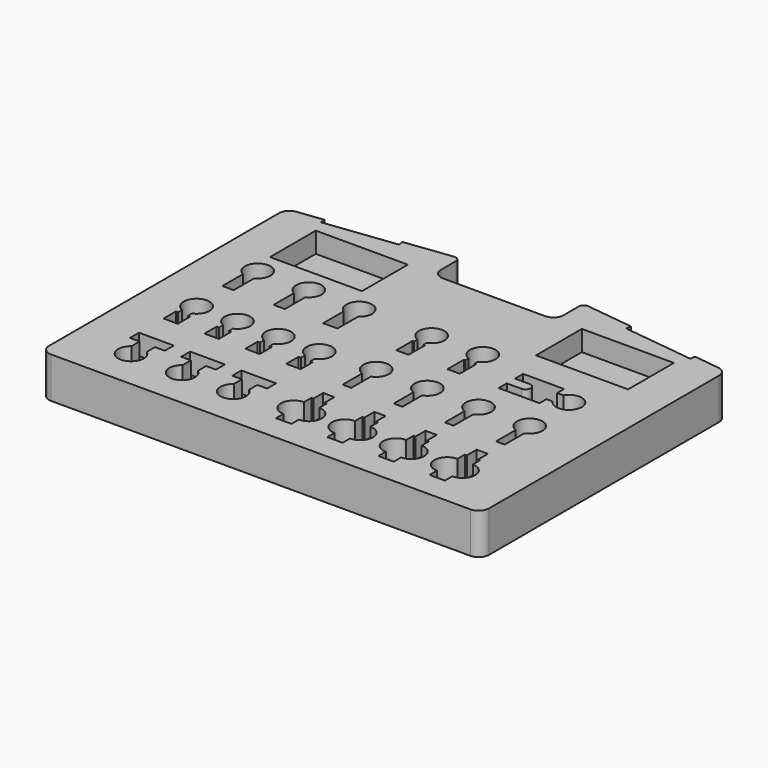
from build123d import *

# Parameters (mm, degrees)
F0_W     = 90
F0_H     = 56
F1_DEPTH = 20
F2_DEPTH = 20


# Not quite as in the source:
# - a feature names something its author has since deleted; it is built from what else it names


with BuildPart() as f1:
    # F0 (on Top) → F1 (new body)
    with BuildSketch(Plane.XY):
        with BuildLine():
            ThreePointArc((0, 10), (2.9289321881, 2.9289321881), (10, 0))
            Line((10, 0), (420, 0))
            ThreePointArc((420, 0), (427.0710678119, 2.9289321881), (430, 10))
            Line((430, 10), (430, 291.1509565045))
            ThreePointArc((430, 291.1509565045), (427.4888915944, 297.7779092497), (421.2166994626, 301.0766626465))
            Line((421.2166994626, 301.0766626465), (396.0936149327, 304.1562665566))
            Line((396.0936149327, 304.1562665566), (395.4852652014, 299.1934134856))
            Line((395.4852652014, 299.1934134856), (326.0053222072, 307.7103097236))
            Line((326.0053222072, 307.7103097236), (326.6136719385, 312.6731627946))
            Line((326.6136719385, 312.6731627946), (280.6083497313, 318.3125248716))
            ThreePointArc((280.6083497313, 318.3125248716), (276.6865236274, 317.0941175978), (275, 313.3496718006))
            Line((275, 313.3496718006), (275, 295))
            ThreePointArc((275, 295), (272.0710678119, 287.9289321881), (265, 285))
            Line((265, 285), (165, 285))
            ThreePointArc((165, 285), (157.9289321881, 287.9289321881), (155, 295))
            Line((155, 295), (155, 313.3496718006))
            ThreePointArc((155, 313.3496718006), (153.3134763726, 317.0941175978), (149.3916502687, 318.3125248716))
            Line((149.3916502687, 318.3125248716), (103.3863280615, 312.6731627946))
            Line((103.3863280615, 312.6731627946), (103.9946777928, 307.7103097236))
            Line((103.9946777928, 307.7103097236), (34.5147347986, 299.1934134856))
            Line((34.5147347986, 299.1934134856), (33.9063850673, 304.1562665566))
            Line((33.9063850673, 304.1562665566), (8.7833005374, 301.0766626465))
            ThreePointArc((8.7833005374, 301.0766626465), (2.5111084056, 297.7779092497), (0, 291.1509565045))
            Line((0, 291.1509565045), (0, 10))
        make_face()
        with BuildLine():
            Line((49.5, 59), (40, 59))
            Line((40, 59), (40, 70))
            Line((40, 70), (74, 70))
            Line((74, 70), (74, 59))
            Line((74, 59), (64.5, 59))
            Line((64.5, 59), (64.5, 49))
            ThreePointArc((64.5, 49), (57, 26.5), (49.5, 49))
            Line((49.5, 49), (49.5, 59))
        make_face(mode=Mode.SUBTRACT)
        with BuildLine():
            Line((99.5, 59), (90, 59))
            Line((90, 59), (90, 70))
            Line((90, 70), (124, 70))
            Line((124, 70), (124, 59))
            Line((124, 59), (114.5, 59))
            Line((114.5, 59), (114.5, 49))
            ThreePointArc((114.5, 49), (107, 26.5), (99.5, 49))
            Line((99.5, 49), (99.5, 59))
        make_face(mode=Mode.SUBTRACT)
        with BuildLine():
            Line((149.5, 59), (140, 59))
            Line((140, 59), (140, 70))
            Line((140, 70), (174, 70))
            Line((174, 70), (174, 59))
            Line((174, 59), (164.5, 59))
            Line((164.5, 59), (164.5, 49))
            ThreePointArc((164.5, 49), (157, 26.5), (149.5, 49))
            Line((149.5, 49), (149.5, 59))
        make_face(mode=Mode.SUBTRACT)
        with BuildLine():
            Line((54, 100), (40, 100))
            Line((40, 100), (40, 115))
            Line((40, 115), (42.25, 115))
            Line((42.25, 115), (42.25, 120))
            ThreePointArc((42.25, 120), (47, 144.0623310798), (51.75, 120))
            Line((51.75, 120), (51.75, 115))
            Line((51.75, 115), (54, 115))
            Line((54, 115), (54, 100))
        make_face(mode=Mode.SUBTRACT)
        with BuildLine():
            Line((94, 100), (80, 100))
            Line((80, 100), (80, 115))
            Line((80, 115), (82.25, 115))
            Line((82.25, 115), (82.25, 120))
            ThreePointArc((82.25, 120), (87, 144.0623310798), (91.75, 120))
            Line((91.75, 120), (91.75, 115))
            Line((91.75, 115), (94, 115))
            Line((94, 115), (94, 100))
        make_face(mode=Mode.SUBTRACT)
        with BuildLine():
            Line((134, 100), (120, 100))
            Line((120, 100), (120, 115))
            Line((120, 115), (122.25, 115))
            Line((122.25, 115), (122.25, 120))
            ThreePointArc((122.25, 120), (127, 144.0623310798), (131.75, 120))
            Line((131.75, 120), (131.75, 115))
            Line((131.75, 115), (134, 115))
            Line((134, 115), (134, 100))
        make_face(mode=Mode.SUBTRACT)
        with BuildLine():
            Line((174, 100), (160, 100))
            Line((160, 100), (160, 115))
            Line((160, 115), (162.25, 115))
            Line((162.25, 115), (162.25, 120))
            ThreePointArc((162.25, 120), (167, 144.0623310798), (171.75, 120))
            Line((171.75, 120), (171.75, 115))
            Line((171.75, 115), (174, 115))
            Line((174, 115), (174, 100))
        make_face(mode=Mode.SUBTRACT)
        with BuildLine():
            Line((225, 25), (210, 25))
            Line((210, 25), (210, 34))
            ThreePointArc((210, 34), (197.5, 46.5), (210, 59))
            Line((210, 59), (210, 68))
            Line((210, 68), (212, 68))
            Line((212, 68), (212, 80))
            Line((212, 80), (223, 80))
            Line((223, 80), (223, 68))
            Line((223, 68), (225, 68))
            Line((225, 68), (225, 59))
            ThreePointArc((225, 59), (237.5, 46.5), (225, 34))
            Line((225, 34), (225, 25))
        make_face(mode=Mode.SUBTRACT)
        with BuildLine():
            Line((275, 34), (275, 25))
            Line((275, 25), (260, 25))
            Line((260, 25), (260, 34))
            ThreePointArc((260, 34), (247.5, 46.5), (260, 59))
            Line((260, 59), (260, 68))
            Line((260, 68), (262, 68))
            Line((262, 68), (262, 80))
            Line((262, 80), (273, 80))
            Line((273, 80), (273, 68))
            Line((273, 68), (275, 68))
            Line((275, 68), (275, 59))
            ThreePointArc((275, 59), (287.5, 46.5), (275, 34))
        make_face(mode=Mode.SUBTRACT)
        with BuildLine():
            Line((325, 34), (325, 25))
            Line((325, 25), (310, 25))
            Line((310, 25), (310, 34))
            ThreePointArc((310, 34), (297.5, 46.5), (310, 59))
            Line((310, 59), (310, 68))
            Line((310, 68), (312, 68))
            Line((312, 68), (312, 80))
            Line((312, 80), (323, 80))
            Line((323, 80), (323, 68))
            Line((323, 68), (325, 68))
            Line((325, 68), (325, 59))
            ThreePointArc((325, 59), (337.5, 46.5), (325, 34))
        make_face(mode=Mode.SUBTRACT)
        with BuildLine():
            Line((375, 34), (375, 25))
            Line((375, 25), (360, 25))
            Line((360, 25), (360, 34))
            ThreePointArc((360, 34), (347.5, 46.5), (360, 59))
            Line((360, 59), (360, 68))
            Line((360, 68), (362, 68))
            Line((362, 68), (362, 80))
            Line((362, 80), (373, 80))
            Line((373, 80), (373, 68))
            Line((373, 68), (375, 68))
            Line((375, 68), (375, 59))
            ThreePointArc((375, 59), (387.5, 46.5), (375, 34))
        make_face(mode=Mode.SUBTRACT)
        with BuildLine():
            Line((223.5, 124), (223.5, 100))
            Line((223.5, 100), (215, 100))
            Line((215, 100), (215, 124))
            ThreePointArc((215, 124), (219.25, 148.2553179455), (223.5, 124))
        make_face(mode=Mode.SUBTRACT)
        with BuildLine():
            Line((273.5, 124), (273.5, 100))
            Line((273.5, 100), (265, 100))
            Line((265, 100), (265, 124))
            ThreePointArc((265, 124), (269.25, 148.2553179455), (273.5, 124))
        make_face(mode=Mode.SUBTRACT)
        with BuildLine():
            Line((323.5, 124), (323.5, 100))
            Line((323.5, 100), (315, 100))
            Line((315, 100), (315, 124))
            ThreePointArc((315, 124), (319.25, 148.2553179455), (323.5, 124))
        make_face(mode=Mode.SUBTRACT)
        with BuildLine():
            Line((373.5, 124), (373.5, 100))
            Line((373.5, 100), (365, 100))
            Line((365, 100), (365, 124))
            ThreePointArc((365, 124), (369.25, 148.2553179455), (373.5, 124))
        make_face(mode=Mode.SUBTRACT)
        with BuildLine():
            Line((52.5, 170), (41.5, 170))
            Line((41.5, 170), (41.5, 195))
            ThreePointArc((41.5, 195), (47, 218.7249721603), (52.5, 195))
            Line((52.5, 195), (52.5, 170))
        make_face(mode=Mode.SUBTRACT)
        with BuildLine():
            Line((102.5, 170), (91.5, 170))
            Line((91.5, 170), (91.5, 195))
            ThreePointArc((91.5, 195), (97, 218.7249721603), (102.5, 195))
            Line((102.5, 195), (102.5, 170))
        make_face(mode=Mode.SUBTRACT)
        with BuildLine():
            Line((154, 170), (140, 170))
            Line((140, 170), (140, 195))
            ThreePointArc((140, 195), (147, 217.8561575886), (154, 195))
            Line((154, 195), (154, 170))
        make_face(mode=Mode.SUBTRACT)
        with Locations((85, 258)):
            Rectangle(F0_W, F0_H, mode=Mode.SUBTRACT)
        with BuildLine():
            Line((223.5, 170), (211.5, 170))
            Line((211.5, 170), (211.5, 190))
            Line((211.5, 190), (213, 190))
            Line((213, 190), (213, 194))
            ThreePointArc((213, 194), (217.5, 218.1619037897), (222, 194))
            Line((222, 194), (222, 190))
            Line((222, 190), (223.5, 190))
            Line((223.5, 190), (223.5, 170))
        make_face(mode=Mode.SUBTRACT)
        with BuildLine():
            Line((273.5, 170), (261.5, 170))
            Line((261.5, 170), (261.5, 190))
            Line((261.5, 190), (263, 190))
            Line((263, 190), (263, 194))
            ThreePointArc((263, 194), (267.5, 218.1619037897), (272, 194))
            Line((272, 194), (272, 190))
            Line((272, 190), (273.5, 190))
            Line((273.5, 190), (273.5, 170))
        make_face(mode=Mode.SUBTRACT)
        with BuildLine():
            Line((351.5, 178.5), (351.5, 170))
            Line((351.5, 170), (311.5, 170))
            Line((311.5, 170), (311.5, 180))
            Line((311.5, 180), (325.8, 180))
            ThreePointArc((325.8, 180), (330.8, 185), (325.8, 190))
            Line((325.8, 190), (311.5, 190))
            Line((311.5, 190), (311.5, 200))
            Line((311.5, 200), (351.5, 200))
            Line((351.5, 200), (351.5, 191.5))
            Line((351.5, 191.5), (357.5, 191.5))
            ThreePointArc((357.5, 191.5), (380.677078252, 185), (357.5, 178.5))
            Line((357.5, 178.5), (351.5, 178.5))
        make_face(mode=Mode.SUBTRACT)
        with Locations((345, 258)):
            Rectangle(F0_W, F0_H, mode=Mode.SUBTRACT)
    extrude(amount=F1_DEPTH)

    # F0 (on Top) → F2 (join)
    with BuildSketch(Plane.XY):
        with BuildLine():
            ThreePointArc((0, 10), (2.9289321881, 2.9289321881), (10, 0))
            Line((10, 0), (420, 0))
            ThreePointArc((420, 0), (427.0710678119, 2.9289321881), (430, 10))
            Line((430, 10), (430, 291.1509565045))
            ThreePointArc((430, 291.1509565045), (427.4888915944, 297.7779092497), (421.2166994626, 301.0766626465))
            Line((421.2166994626, 301.0766626465), (396.0936149327, 304.1562665566))
            Line((396.0936149327, 304.1562665566), (395.4852652014, 299.1934134856))
            Line((395.4852652014, 299.1934134856), (326.0053222072, 307.7103097236))
            Line((326.0053222072, 307.7103097236), (326.6136719385, 312.6731627946))
            Line((326.6136719385, 312.6731627946), (280.6083497313, 318.3125248716))
            ThreePointArc((280.6083497313, 318.3125248716), (276.6865236274, 317.0941175978), (275, 313.3496718006))
            Line((275, 313.3496718006), (275, 295))
            ThreePointArc((275, 295), (272.0710678119, 287.9289321881), (265, 285))
            Line((265, 285), (165, 285))
            ThreePointArc((165, 285), (157.9289321881, 287.9289321881), (155, 295))
            Line((155, 295), (155, 313.3496718006))
            ThreePointArc((155, 313.3496718006), (153.3134763726, 317.0941175978), (149.3916502687, 318.3125248716))
            Line((149.3916502687, 318.3125248716), (103.3863280615, 312.6731627946))
            Line((103.3863280615, 312.6731627946), (103.9946777928, 307.7103097236))
            Line((103.9946777928, 307.7103097236), (34.5147347986, 299.1934134856))
            Line((34.5147347986, 299.1934134856), (33.9063850673, 304.1562665566))
            Line((33.9063850673, 304.1562665566), (8.7833005374, 301.0766626465))
            ThreePointArc((8.7833005374, 301.0766626465), (2.5111084056, 297.7779092497), (0, 291.1509565045))
            Line((0, 291.1509565045), (0, 10))
        make_face()
        with BuildLine():
            Line((49.5, 59), (40, 59))
            Line((40, 59), (40, 70))
            Line((40, 70), (74, 70))
            Line((74, 70), (74, 59))
            Line((74, 59), (64.5, 59))
            Line((64.5, 59), (64.5, 49))
            ThreePointArc((64.5, 49), (57, 26.5), (49.5, 49))
            Line((49.5, 49), (49.5, 59))
        make_face(mode=Mode.SUBTRACT)
        with BuildLine():
            Line((99.5, 59), (90, 59))
            Line((90, 59), (90, 70))
            Line((90, 70), (124, 70))
            Line((124, 70), (124, 59))
            Line((124, 59), (114.5, 59))
            Line((114.5, 59), (114.5, 49))
            ThreePointArc((114.5, 49), (107, 26.5), (99.5, 49))
            Line((99.5, 49), (99.5, 59))
        make_face(mode=Mode.SUBTRACT)
        with BuildLine():
            Line((149.5, 59), (140, 59))
            Line((140, 59), (140, 70))
            Line((140, 70), (174, 70))
            Line((174, 70), (174, 59))
            Line((174, 59), (164.5, 59))
            Line((164.5, 59), (164.5, 49))
            ThreePointArc((164.5, 49), (157, 26.5), (149.5, 49))
            Line((149.5, 49), (149.5, 59))
        make_face(mode=Mode.SUBTRACT)
        with BuildLine():
            Line((54, 100), (40, 100))
            Line((40, 100), (40, 115))
            Line((40, 115), (42.25, 115))
            Line((42.25, 115), (42.25, 120))
            ThreePointArc((42.25, 120), (47, 144.0623310798), (51.75, 120))
            Line((51.75, 120), (51.75, 115))
            Line((51.75, 115), (54, 115))
            Line((54, 115), (54, 100))
        make_face(mode=Mode.SUBTRACT)
        with BuildLine():
            Line((94, 100), (80, 100))
            Line((80, 100), (80, 115))
            Line((80, 115), (82.25, 115))
            Line((82.25, 115), (82.25, 120))
            ThreePointArc((82.25, 120), (87, 144.0623310798), (91.75, 120))
            Line((91.75, 120), (91.75, 115))
            Line((91.75, 115), (94, 115))
            Line((94, 115), (94, 100))
        make_face(mode=Mode.SUBTRACT)
        with BuildLine():
            Line((134, 100), (120, 100))
            Line((120, 100), (120, 115))
            Line((120, 115), (122.25, 115))
            Line((122.25, 115), (122.25, 120))
            ThreePointArc((122.25, 120), (127, 144.0623310798), (131.75, 120))
            Line((131.75, 120), (131.75, 115))
            Line((131.75, 115), (134, 115))
            Line((134, 115), (134, 100))
        make_face(mode=Mode.SUBTRACT)
        with BuildLine():
            Line((174, 100), (160, 100))
            Line((160, 100), (160, 115))
            Line((160, 115), (162.25, 115))
            Line((162.25, 115), (162.25, 120))
            ThreePointArc((162.25, 120), (167, 144.0623310798), (171.75, 120))
            Line((171.75, 120), (171.75, 115))
            Line((171.75, 115), (174, 115))
            Line((174, 115), (174, 100))
        make_face(mode=Mode.SUBTRACT)
        with BuildLine():
            Line((225, 25), (210, 25))
            Line((210, 25), (210, 34))
            ThreePointArc((210, 34), (197.5, 46.5), (210, 59))
            Line((210, 59), (210, 68))
            Line((210, 68), (212, 68))
            Line((212, 68), (212, 80))
            Line((212, 80), (223, 80))
            Line((223, 80), (223, 68))
            Line((223, 68), (225, 68))
            Line((225, 68), (225, 59))
            ThreePointArc((225, 59), (237.5, 46.5), (225, 34))
            Line((225, 34), (225, 25))
        make_face(mode=Mode.SUBTRACT)
        with BuildLine():
            Line((275, 34), (275, 25))
            Line((275, 25), (260, 25))
            Line((260, 25), (260, 34))
            ThreePointArc((260, 34), (247.5, 46.5), (260, 59))
            Line((260, 59), (260, 68))
            Line((260, 68), (262, 68))
            Line((262, 68), (262, 80))
            Line((262, 80), (273, 80))
            Line((273, 80), (273, 68))
            Line((273, 68), (275, 68))
            Line((275, 68), (275, 59))
            ThreePointArc((275, 59), (287.5, 46.5), (275, 34))
        make_face(mode=Mode.SUBTRACT)
        with BuildLine():
            Line((325, 34), (325, 25))
            Line((325, 25), (310, 25))
            Line((310, 25), (310, 34))
            ThreePointArc((310, 34), (297.5, 46.5), (310, 59))
            Line((310, 59), (310, 68))
            Line((310, 68), (312, 68))
            Line((312, 68), (312, 80))
            Line((312, 80), (323, 80))
            Line((323, 80), (323, 68))
            Line((323, 68), (325, 68))
            Line((325, 68), (325, 59))
            ThreePointArc((325, 59), (337.5, 46.5), (325, 34))
        make_face(mode=Mode.SUBTRACT)
        with BuildLine():
            Line((375, 34), (375, 25))
            Line((375, 25), (360, 25))
            Line((360, 25), (360, 34))
            ThreePointArc((360, 34), (347.5, 46.5), (360, 59))
            Line((360, 59), (360, 68))
            Line((360, 68), (362, 68))
            Line((362, 68), (362, 80))
            Line((362, 80), (373, 80))
            Line((373, 80), (373, 68))
            Line((373, 68), (375, 68))
            Line((375, 68), (375, 59))
            ThreePointArc((375, 59), (387.5, 46.5), (375, 34))
        make_face(mode=Mode.SUBTRACT)
        with BuildLine():
            Line((223.5, 124), (223.5, 100))
            Line((223.5, 100), (215, 100))
            Line((215, 100), (215, 124))
            ThreePointArc((215, 124), (219.25, 148.2553179455), (223.5, 124))
        make_face(mode=Mode.SUBTRACT)
        with BuildLine():
            Line((273.5, 124), (273.5, 100))
            Line((273.5, 100), (265, 100))
            Line((265, 100), (265, 124))
            ThreePointArc((265, 124), (269.25, 148.2553179455), (273.5, 124))
        make_face(mode=Mode.SUBTRACT)
        with BuildLine():
            Line((323.5, 124), (323.5, 100))
            Line((323.5, 100), (315, 100))
            Line((315, 100), (315, 124))
            ThreePointArc((315, 124), (319.25, 148.2553179455), (323.5, 124))
        make_face(mode=Mode.SUBTRACT)
        with BuildLine():
            Line((373.5, 124), (373.5, 100))
            Line((373.5, 100), (365, 100))
            Line((365, 100), (365, 124))
            ThreePointArc((365, 124), (369.25, 148.2553179455), (373.5, 124))
        make_face(mode=Mode.SUBTRACT)
        with BuildLine():
            Line((52.5, 170), (41.5, 170))
            Line((41.5, 170), (41.5, 195))
            ThreePointArc((41.5, 195), (47, 218.7249721603), (52.5, 195))
            Line((52.5, 195), (52.5, 170))
        make_face(mode=Mode.SUBTRACT)
        with BuildLine():
            Line((102.5, 170), (91.5, 170))
            Line((91.5, 170), (91.5, 195))
            ThreePointArc((91.5, 195), (97, 218.7249721603), (102.5, 195))
            Line((102.5, 195), (102.5, 170))
        make_face(mode=Mode.SUBTRACT)
        with BuildLine():
            Line((154, 170), (140, 170))
            Line((140, 170), (140, 195))
            ThreePointArc((140, 195), (147, 217.8561575886), (154, 195))
            Line((154, 195), (154, 170))
        make_face(mode=Mode.SUBTRACT)
        with Locations((85, 258)):
            Rectangle(F0_W, F0_H, mode=Mode.SUBTRACT)
        with BuildLine():
            Line((223.5, 170), (211.5, 170))
            Line((211.5, 170), (211.5, 190))
            Line((211.5, 190), (213, 190))
            Line((213, 190), (213, 194))
            ThreePointArc((213, 194), (217.5, 218.1619037897), (222, 194))
            Line((222, 194), (222, 190))
            Line((222, 190), (223.5, 190))
            Line((223.5, 190), (223.5, 170))
        make_face(mode=Mode.SUBTRACT)
        with BuildLine():
            Line((273.5, 170), (261.5, 170))
            Line((261.5, 170), (261.5, 190))
            Line((261.5, 190), (263, 190))
            Line((263, 190), (263, 194))
            ThreePointArc((263, 194), (267.5, 218.1619037897), (272, 194))
            Line((272, 194), (272, 190))
            Line((272, 190), (273.5, 190))
            Line((273.5, 190), (273.5, 170))
        make_face(mode=Mode.SUBTRACT)
        with BuildLine():
            Line((351.5, 178.5), (351.5, 170))
            Line((351.5, 170), (311.5, 170))
            Line((311.5, 170), (311.5, 180))
            Line((311.5, 180), (325.8, 180))
            ThreePointArc((325.8, 180), (330.8, 185), (325.8, 190))
            Line((325.8, 190), (311.5, 190))
            Line((311.5, 190), (311.5, 200))
            Line((311.5, 200), (351.5, 200))
            Line((351.5, 200), (351.5, 191.5))
            Line((351.5, 191.5), (357.5, 191.5))
            ThreePointArc((357.5, 191.5), (380.677078252, 185), (357.5, 178.5))
            Line((357.5, 178.5), (351.5, 178.5))
        make_face(mode=Mode.SUBTRACT)
        with Locations((345, 258)):
            Rectangle(F0_W, F0_H, mode=Mode.SUBTRACT)
        with Locations((85, 258)):
            Rectangle(F0_W, F0_H)
        with Locations((345, 258)):
            Rectangle(F0_W, F0_H)
        with BuildLine():
            Line((311.5, 170), (351.5, 170))
            Line((351.5, 170), (351.5, 178.5))
            Line((351.5, 178.5), (357.5, 178.5))
            ThreePointArc((357.5, 178.5), (380.677078252, 185), (357.5, 191.5))
            Line((357.5, 191.5), (351.5, 191.5))
            Line((351.5, 191.5), (351.5, 200))
            Line((351.5, 200), (311.5, 200))
            Line((311.5, 200), (311.5, 190))
            Line((311.5, 190), (325.8, 190))
            ThreePointArc((325.8, 190), (330.8, 185), (325.8, 180))
            Line((325.8, 180), (311.5, 180))
            Line((311.5, 180), (311.5, 170))
        make_face()
        with BuildLine():
            Line((261.5, 190), (261.5, 170))
            Line((261.5, 170), (273.5, 170))
            Line((273.5, 170), (273.5, 190))
            Line((273.5, 190), (272, 190))
            Line((272, 190), (272, 194))
            ThreePointArc((272, 194), (267.5, 218.1619037897), (263, 194))
            Line((263, 194), (263, 190))
            Line((263, 190), (261.5, 190))
        make_face()
        with BuildLine():
            Line((211.5, 190), (211.5, 170))
            Line((211.5, 170), (223.5, 170))
            Line((223.5, 170), (223.5, 190))
            Line((223.5, 190), (222, 190))
            Line((222, 190), (222, 194))
            ThreePointArc((222, 194), (217.5, 218.1619037897), (213, 194))
            Line((213, 194), (213, 190))
            Line((213, 190), (211.5, 190))
        make_face()
        with BuildLine():
            Line((140, 195), (140, 170))
            Line((140, 170), (154, 170))
            Line((154, 170), (154, 195))
            ThreePointArc((154, 195), (147, 217.8561575886), (140, 195))
        make_face()
        with BuildLine():
            Line((91.5, 195), (91.5, 170))
            Line((91.5, 170), (102.5, 170))
            Line((102.5, 170), (102.5, 195))
            ThreePointArc((102.5, 195), (97, 218.7249721603), (91.5, 195))
        make_face()
        with BuildLine():
            Line((41.5, 195), (41.5, 170))
            Line((41.5, 170), (52.5, 170))
            Line((52.5, 170), (52.5, 195))
            ThreePointArc((52.5, 195), (47, 218.7249721603), (41.5, 195))
        make_face()
        with BuildLine():
            Line((40, 115), (40, 100))
            Line((40, 100), (54, 100))
            Line((54, 100), (54, 115))
            Line((54, 115), (51.75, 115))
            Line((51.75, 115), (51.75, 120))
            ThreePointArc((51.75, 120), (47, 144.0623310798), (42.25, 120))
            Line((42.25, 120), (42.25, 115))
            Line((42.25, 115), (40, 115))
        make_face()
        with BuildLine():
            Line((80, 115), (80, 100))
            Line((80, 100), (94, 100))
            Line((94, 100), (94, 115))
            Line((94, 115), (91.75, 115))
            Line((91.75, 115), (91.75, 120))
            ThreePointArc((91.75, 120), (87, 144.0623310798), (82.25, 120))
            Line((82.25, 120), (82.25, 115))
            Line((82.25, 115), (80, 115))
        make_face()
        with BuildLine():
            Line((120, 115), (120, 100))
            Line((120, 100), (134, 100))
            Line((134, 100), (134, 115))
            Line((134, 115), (131.75, 115))
            Line((131.75, 115), (131.75, 120))
            ThreePointArc((131.75, 120), (127, 144.0623310798), (122.25, 120))
            Line((122.25, 120), (122.25, 115))
            Line((122.25, 115), (120, 115))
        make_face()
        with BuildLine():
            Line((160, 115), (160, 100))
            Line((160, 100), (174, 100))
            Line((174, 100), (174, 115))
            Line((174, 115), (171.75, 115))
            Line((171.75, 115), (171.75, 120))
            ThreePointArc((171.75, 120), (167, 144.0623310798), (162.25, 120))
            Line((162.25, 120), (162.25, 115))
            Line((162.25, 115), (160, 115))
        make_face()
        with BuildLine():
            Line((215, 100), (223.5, 100))
            Line((223.5, 100), (223.5, 124))
            ThreePointArc((223.5, 124), (219.25, 148.2553179455), (215, 124))
            Line((215, 124), (215, 100))
        make_face()
        with BuildLine():
            Line((265, 100), (273.5, 100))
            Line((273.5, 100), (273.5, 124))
            ThreePointArc((273.5, 124), (269.25, 148.2553179455), (265, 124))
            Line((265, 124), (265, 100))
        make_face()
        with BuildLine():
            Line((315, 100), (323.5, 100))
            Line((323.5, 100), (323.5, 124))
            ThreePointArc((323.5, 124), (319.25, 148.2553179455), (315, 124))
            Line((315, 124), (315, 100))
        make_face()
        with BuildLine():
            Line((365, 100), (373.5, 100))
            Line((373.5, 100), (373.5, 124))
            ThreePointArc((373.5, 124), (369.25, 148.2553179455), (365, 124))
            Line((365, 124), (365, 100))
        make_face()
        with BuildLine():
            Line((360, 25), (375, 25))
            Line((375, 25), (375, 34))
            ThreePointArc((375, 34), (387.5, 46.5), (375, 59))
            Line((375, 59), (375, 68))
            Line((375, 68), (373, 68))
            Line((373, 68), (373, 80))
            Line((373, 80), (362, 80))
            Line((362, 80), (362, 68))
            Line((362, 68), (360, 68))
            Line((360, 68), (360, 59))
            ThreePointArc((360, 59), (347.5, 46.5), (360, 34))
            Line((360, 34), (360, 25))
        make_face()
        with BuildLine():
            Line((310, 25), (325, 25))
            Line((325, 25), (325, 34))
            ThreePointArc((325, 34), (337.5, 46.5), (325, 59))
            Line((325, 59), (325, 68))
            Line((325, 68), (323, 68))
            Line((323, 68), (323, 80))
            Line((323, 80), (312, 80))
            Line((312, 80), (312, 68))
            Line((312, 68), (310, 68))
            Line((310, 68), (310, 59))
            ThreePointArc((310, 59), (297.5, 46.5), (310, 34))
            Line((310, 34), (310, 25))
        make_face()
        with BuildLine():
            Line((260, 25), (275, 25))
            Line((275, 25), (275, 34))
            ThreePointArc((275, 34), (287.5, 46.5), (275, 59))
            Line((275, 59), (275, 68))
            Line((275, 68), (273, 68))
            Line((273, 68), (273, 80))
            Line((273, 80), (262, 80))
            Line((262, 80), (262, 68))
            Line((262, 68), (260, 68))
            Line((260, 68), (260, 59))
            ThreePointArc((260, 59), (247.5, 46.5), (260, 34))
            Line((260, 34), (260, 25))
        make_face()
        with BuildLine():
            Line((210, 34), (210, 25))
            Line((210, 25), (225, 25))
            Line((225, 25), (225, 34))
            ThreePointArc((225, 34), (237.5, 46.5), (225, 59))
            Line((225, 59), (225, 68))
            Line((225, 68), (223, 68))
            Line((223, 68), (223, 80))
            Line((223, 80), (212, 80))
            Line((212, 80), (212, 68))
            Line((212, 68), (210, 68))
            Line((210, 68), (210, 59))
            ThreePointArc((210, 59), (197.5, 46.5), (210, 34))
        make_face()
        with BuildLine():
            Line((140, 70), (140, 59))
            Line((140, 59), (149.5, 59))
            Line((149.5, 59), (149.5, 49))
            ThreePointArc((149.5, 49), (157, 26.5), (164.5, 49))
            Line((164.5, 49), (164.5, 59))
            Line((164.5, 59), (174, 59))
            Line((174, 59), (174, 70))
            Line((174, 70), (140, 70))
        make_face()
        with BuildLine():
            Line((90, 70), (90, 59))
            Line((90, 59), (99.5, 59))
            Line((99.5, 59), (99.5, 49))
            ThreePointArc((99.5, 49), (107, 26.5), (114.5, 49))
            Line((114.5, 49), (114.5, 59))
            Line((114.5, 59), (124, 59))
            Line((124, 59), (124, 70))
            Line((124, 70), (90, 70))
        make_face()
        with BuildLine():
            Line((40, 70), (40, 59))
            Line((40, 59), (49.5, 59))
            Line((49.5, 59), (49.5, 49))
            ThreePointArc((49.5, 49), (57, 26.5), (64.5, 49))
            Line((64.5, 49), (64.5, 59))
            Line((64.5, 59), (74, 59))
            Line((74, 59), (74, 70))
            Line((74, 70), (40, 70))
        make_face()
    extrude(amount=-F2_DEPTH)


solid = f1.part
